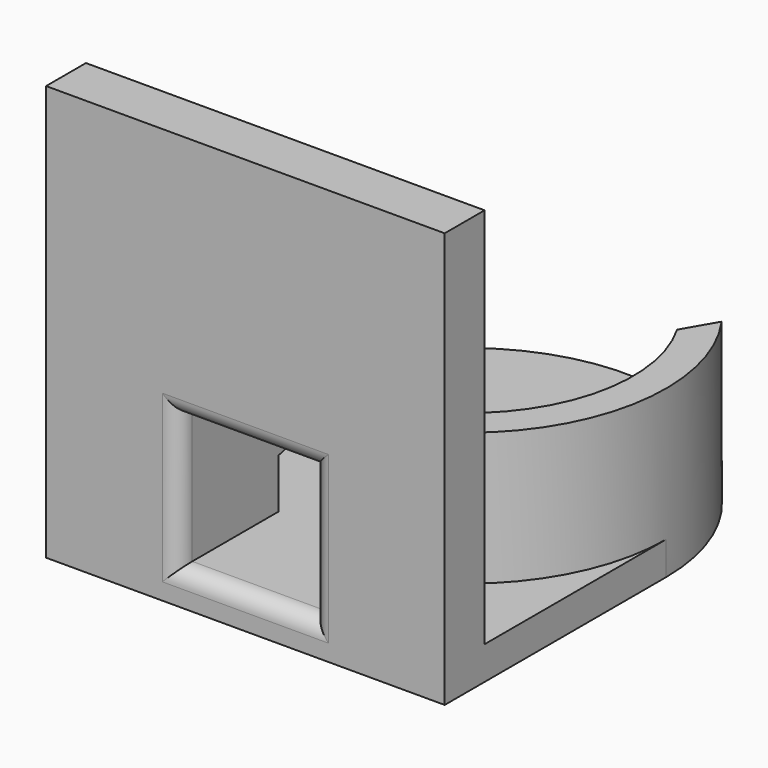
from build123d import *

# Parameters (mm, degrees)
F1_DEPTH  = 2
F3_DEPTH  = 3
F5_DEPTH  = 2
F7_DEPTH  = 3
F8_R      = 0.99999
F9_W      = 24
F9_H      = 22.6653645039
F10_DEPTH = 10
F11_W     = 24
F11_H     = 25
F11_W_2   = 8
F11_H_2   = 8
F12_DEPTH = 3
F13_R     = 1
F14_W     = 24
F14_H     = 13.6653645039
F15_DEPTH = 2


# Not quite as in the source:
# - a fillet or chamfer is up to 0.001 mm smaller than in the source, because OpenCascade refuses the exact size


with BuildPart() as f1:
    # F0 (on Top) → F1 (new body)
    with BuildSketch(Plane.XY):
        with BuildLine():
            ThreePointArc((5.5, 1.5), (0, 24.1653645039), (-5.5, 1.5))
            Line((-5.5, 1.5), (-5.5, -1.5))
            ThreePointArc((-5.5, -1.5), (0, -24.1653645039), (5.5, -1.5))
            Line((5.5, -1.5), (5.5, 1.5))
        make_face()
    extrude(amount=F1_DEPTH)

    # F2 (on face) → F3 (join)
    with BuildSketch(Plane.XY.offset(2)):
        with BuildLine():
            Line((9.7844830762, 19.1125863177), (8.6602540378, 17.1653645039))
            ThreePointArc((8.6602540378, 17.1653645039), (9.4991255677, 9.0402063559), (4, 3.0002131139))
            Line((4, 3.0002131139), (4, -6.2432010007))
            Line((4, -6.2432010007), (9.1651513899, -16.1653645039))
            ThreePointArc((9.1651513899, -16.1653645039), (9.5868378212, -9.3206253964), (5.5, -3.8137179596))
            Line((5.5, -3.8137179596), (5.5, 1.5))
            ThreePointArc((5.5, 1.5), (11.6599594736, 9.3289327537), (9.7844830762, 19.1125863177))
        make_face()
        with BuildLine():
            ThreePointArc((-4, 3.0002131139), (-9.4991255677, 9.0402063559), (-8.6602540378, 17.1653645039))
            Line((-8.6602540378, 17.1653645039), (-9.7844830762, 19.1125863177))
            ThreePointArc((-9.7844830762, 19.1125863177), (-11.6599594736, 9.3289327537), (-5.5, 1.5))
            Line((-5.5, 1.5), (-5.5, -3.8137179596))
            ThreePointArc((-5.5, -3.8137179596), (-9.5868378212, -9.3206253964), (-9.1651513899, -16.1653645039))
            Line((-9.1651513899, -16.1653645039), (-4, -6.2432010007))
            Line((-4, -6.2432010007), (-4, 3.0002131139))
        make_face()
    extrude(amount=F3_DEPTH)

    # F4 (on face) → F5 (join)
    with BuildSketch(Plane.XY.offset(5)):
        with BuildLine():
            Line((-8.0717844057, 16.1461052023), (-9.7844830762, 19.1125863177))
            ThreePointArc((-9.7844830762, 19.1125863177), (-11.6599594736, 9.3289327537), (-5.5, 1.5))
            Line((-5.5, 1.5), (-5.5, -5.0414610795))
            ThreePointArc((-5.5, -5.0414610795), (-8.6043935433, -9.5263473097), (-8.5483759414, -14.980549891))
            Line((-8.5483759414, -14.980549891), (-4, -6.2432010007))
            Line((-4, -6.2432010007), (-4, 4.1031067556))
            ThreePointArc((-4, 4.1031067556), (-8.5258693153, 9.2827350759), (-8.0717844057, 16.1461052023))
        make_face()
        with BuildLine():
            ThreePointArc((5.5, 1.5), (11.6599594736, 9.3289327537), (9.7844830762, 19.1125863177))
            Line((9.7844830762, 19.1125863177), (8.0717844057, 16.1461052023))
            ThreePointArc((8.0717844057, 16.1461052023), (8.5258693153, 9.2827350759), (4, 4.1031067556))
            Line((4, 4.1031067556), (4, -6.2432010007))
            Line((4, -6.2432010007), (8.5483759414, -14.980549891))
            ThreePointArc((8.5483759414, -14.980549891), (8.6043935433, -9.5263473097), (5.5, -5.0414610795))
            Line((5.5, -5.0414610795), (5.5, 1.5))
        make_face()
    extrude(amount=F5_DEPTH)

    # F6 (on face) → F7 (join)
    with BuildSketch(Plane.XY.offset(7)):
        with BuildLine():
            Line((9.7844830762, 19.1125863177), (8.6602540378, 17.1653645039))
            ThreePointArc((8.6602540378, 17.1653645039), (9.4991255677, 9.0402063559), (4, 3.0002131139))
            Line((4, 3.0002131139), (4, -6.2432010007))
            Line((4, -6.2432010007), (9.1651513899, -16.1653645039))
            ThreePointArc((9.1651513899, -16.1653645039), (9.5868378212, -9.3206253964), (5.5, -3.8137179596))
            Line((5.5, -3.8137179596), (5.5, 1.5))
            ThreePointArc((5.5, 1.5), (11.6599594736, 9.3289327537), (9.7844830762, 19.1125863177))
        make_face()
        with BuildLine():
            ThreePointArc((-4, 3.0002131139), (-9.4991255677, 9.0402063559), (-8.6602540378, 17.1653645039))
            Line((-8.6602540378, 17.1653645039), (-9.7844830762, 19.1125863177))
            ThreePointArc((-9.7844830762, 19.1125863177), (-11.6599594736, 9.3289327537), (-5.5, 1.5))
            Line((-5.5, 1.5), (-5.5, -3.8137179596))
            ThreePointArc((-5.5, -3.8137179596), (-9.5868378212, -9.3206253964), (-9.1651513899, -16.1653645039))
            Line((-9.1651513899, -16.1653645039), (-4, -6.2432010007))
            Line((-4, -6.2432010007), (-4, 3.0002131139))
        make_face()
    extrude(amount=F7_DEPTH)

    # F8 (radius 1 in the source; OpenCascade refuses exactly that, so slightly less here)
    f8_edges = [f1.edges().sort_by_distance(p)[0] for p in [
        (8.525869, 9.282735, 7),
        (-8.525869, 9.282735, 7),
        (-8.525869, 9.282735, 5),
        (8.525869, 9.282735, 5),
        (-8.604394, -9.526347, 5),
        (-8.604394, -9.526347, 7),
        (8.604394, -9.526347, 7),
        (8.604394, -9.526347, 5),
    ]]
    fillet(f8_edges, radius=F8_R)

    # F9 (on face) → F10 (cut)
    with BuildSketch(Plane.XY.offset(10)):
        with Locations((0, -12.8326822519)):
            Rectangle(F9_W, F9_H)
    extrude(amount=-F10_DEPTH, mode=Mode.SUBTRACT)

    # F11 (on face) → F12 (join)
    with BuildSketch(Plane.XZ.offset(1.5)):
        with Locations((0, 12.5)):
            Rectangle(F11_W, F11_H)
        with Locations((0, 6)):
            Rectangle(F11_W_2, F11_H_2, mode=Mode.SUBTRACT)
    extrude(amount=F12_DEPTH)

    # F13
    f13_edges = [f1.edges().sort_by_distance(p)[0] for p in [
        (0, -4.5, 10),
        (4, -4.5, 6),
        (0, -4.5, 2),
        (-4, -4.5, 6),
    ]]
    fillet(f13_edges, radius=F13_R)

    # F14 (on face) → F15 (join)
    with BuildSketch(Plane(origin=(0, 0, 0), x_dir=(1, 0, 0), z_dir=(0, 0, -1))):
        with Locations((0, -5.3326822519)):
            Rectangle(F14_W, F14_H)
    extrude(amount=-F15_DEPTH)


solid = f1.part
